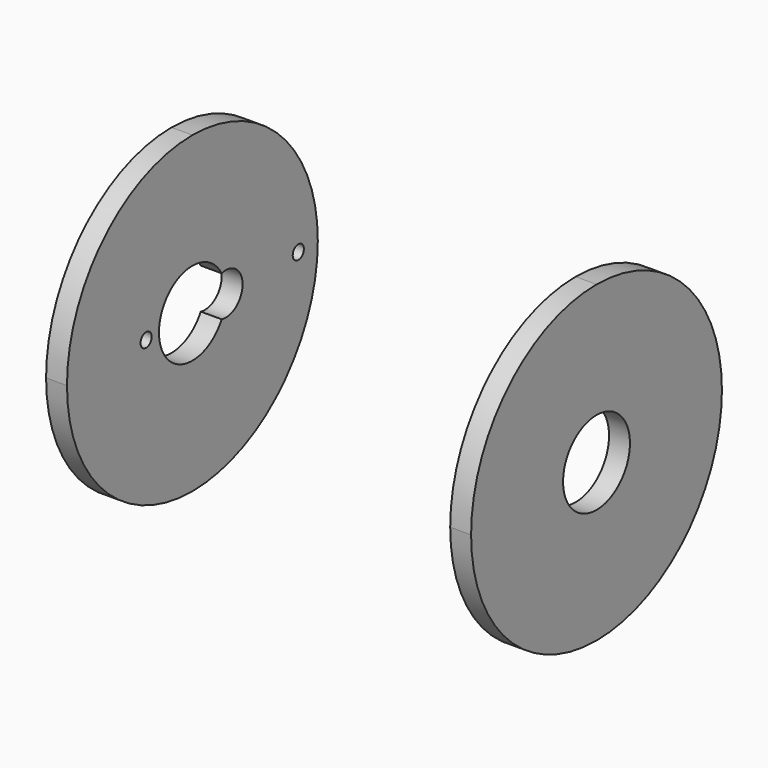
from build123d import *

# Parameters (mm, degrees)
F1_W     = 3
F1_H     = 45
F2_DEPTH = 45
F3_R     = 22.49999
F4_R     = 22.49999
F6_D     = 12
F7_D     = 12
F8_D     = 6
F9_D     = 2


# Not quite as in the source:
# - a fillet or chamfer is up to 0.001 mm smaller than in the source, because OpenCascade refuses the exact size


with BuildPart() as f2:
    # F1 (on Front) → F2 (new body)
    with BuildSketch(Plane.XZ):
        with Locations((-29, 0)):
            Rectangle(F1_W, F1_H)
    extrude(amount=F2_DEPTH)

    # F3 (radius 22.5 in the source; OpenCascade refuses exactly that, so slightly less here)
    f3_edges = [f2.edges().sort_by_distance(p)[0] for p in [
        (-29, -45, 22.5),
        (-29, -45, -22.5),
        (-29, 0, -22.5),
        (-29, 0, 22.5),
    ]]
    fillet(f3_edges, radius=F3_R)

    # F7 (through all)
    with Locations(Plane.YZ):
        with Locations((-22.5, 0)):
            Hole(F7_D / 2)

    # F8 (through all)
    with Locations(Plane.YZ):
        with Locations((-16.5, 0)):
            Hole(F8_D / 2)

    # F9 (through all)
    with Locations(Plane.YZ):
        with Locations((-3.5, 0), (-30.8, 0)):
            Hole(F9_D / 2)


with BuildPart() as f2b:
    # F1 (on Front) → F2, piece 2 (new body)
    with BuildSketch(Plane.XZ):
        with Locations((29, 0)):
            Rectangle(F1_W, F1_H)
    extrude(amount=F2_DEPTH)

    # F4 (radius 22.5 in the source; OpenCascade refuses exactly that, so slightly less here)
    f4_edges = [f2b.edges().sort_by_distance(p)[0] for p in [
        (29, -45, -22.5),
        (29, 0, -22.5),
        (29, 0, 22.5),
        (29, -45, 22.5),
    ]]
    fillet(f4_edges, radius=F4_R)

    # F6 (through all)
    with Locations(Plane(origin=(0, 0, 0), x_dir=(0, 1, 0), z_dir=(-1, 0, 0))):
        with Locations((-22.5, 0)):
            Hole(F6_D / 2)


solid = Compound([f2.part, f2b.part])
